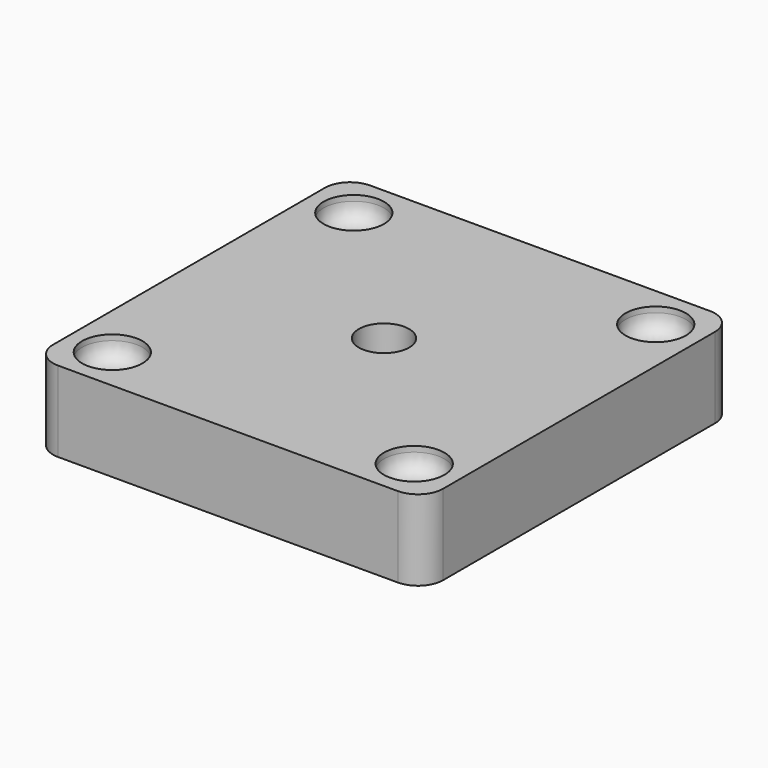
from build123d import *

# Parameters (mm, degrees)
F0_W         = 77.51
F0_H         = 77.519
F0_R         = 2.55
F0_R_2       = 5
F1_DEPTH     = 16
F2_DEPTH     = 7
F3_R         = 5
F4_R         = 6
F4_R_2       = 2.55
F5_DEPTH     = 4.6
F6_S5_R      = 2.55
F6_T6_DEPTH  = 10
F6_S11_R     = 2.55
F6_T12_DEPTH = 10
F6_S17_R     = 2.55
F6_T18_DEPTH = 10
F6_S23_R     = 2.55
F6_T24_DEPTH = 10


# Not quite as in the source:
# - a fillet or chamfer that OpenCascade refuses, or shapes differently, is made with other operations: its cross-section is extruded or revolved along the edge and cut away or added
# - a feature names something its author has since deleted; it is built from what else it names


with BuildPart() as f1:
    # F0 (on Top) → F1 (new body)
    with BuildSketch(Plane.XY):
        Rectangle(F0_W, F0_H)
        with Locations((-30, -29.9995)):
            Circle(F0_R, mode=Mode.SUBTRACT)
        with Locations((30, -29.9995)):
            Circle(F0_R, mode=Mode.SUBTRACT)
        with Locations((-30, 29.9995)):
            Circle(F0_R, mode=Mode.SUBTRACT)
        Polygon((7.25, -4.1857894516), (0, -8.3715789032), (-7.25, -4.1857894516), (-7.25, 4.1857894516), (0, 8.3715789032), (7.25, 4.1857894516), align=None, mode=Mode.SUBTRACT)
        with Locations((30, 29.9995)):
            Circle(F0_R, mode=Mode.SUBTRACT)
        Polygon((-7.25, -4.1857894516), (0, -8.3715789032), (7.25, -4.1857894516), (7.25, 4.1857894516), (0, 8.3715789032), (-7.25, 4.1857894516), align=None)
        Circle(F0_R_2, mode=Mode.SUBTRACT)
    extrude(amount=F1_DEPTH)

    # F0 (on Top) → F2 (cut)
    with BuildSketch(Plane.XY):
        Polygon((-7.25, -4.1857894516), (0, -8.3715789032), (7.25, -4.1857894516), (7.25, 4.1857894516), (0, 8.3715789032), (-7.25, 4.1857894516), align=None)
        Circle(F0_R_2, mode=Mode.SUBTRACT)
    extrude(amount=F2_DEPTH, mode=Mode.SUBTRACT)

    # F3
    f3_edges = [f1.edges().sort_by_distance(p)[0] for p in [
        (38.755, -38.7595, 8),
        (-38.755, -38.7595, 8),
        (38.755, 38.7595, 8),
        (-38.755, 38.7595, 8),
    ]]
    fillet(f3_edges, radius=F3_R)

    # F4 (on face) → F5 (cut)
    with BuildSketch(Plane.XY.offset(16)):
        with Locations((-30, 29.9995)):
            Circle(F4_R)
        with Locations((-30, 29.9995)):
            Circle(F4_R_2, mode=Mode.SUBTRACT)
        with Locations((30, 29.9995)):
            Circle(F4_R)
        with Locations((30, 29.9995)):
            Circle(F4_R_2, mode=Mode.SUBTRACT)
        with Locations((30, -29.9995)):
            Circle(F4_R)
        with Locations((30, -29.9995)):
            Circle(F4_R_2, mode=Mode.SUBTRACT)
        with Locations((-30, -29.9995)):
            Circle(F4_R)
        with Locations((-30, -29.9995)):
            Circle(F4_R_2, mode=Mode.SUBTRACT)
    extrude(amount=-F5_DEPTH, mode=Mode.SUBTRACT)

    # F6: fillet of radius 3.5 on 4 edges, made by hand


with BuildPart() as f6_tool2:
    # F6_s3 → F6_t4 (revolve)
    with BuildSketch(Plane.XZ.offset(29.9995)):
        with BuildLine():
            ThreePointArc((-24, 14.9), (-25.0251262658, 12.4251262658), (-27.5, 11.4))
            Line((-27.5, 11.4), (-24, 11.4))
            Line((-24, 11.4), (-24, 14.9))
        make_face()
    revolve(axis=Axis((-30, -29.9995, 11.4), (0, 0, 1)))

    # F6_s5 → F6_t6 (cut, symmetric)
    with BuildSketch(Plane.XY.offset(13.2)):
        with Locations((-30, -29.9995)):
            Circle(F6_S5_R)
    extrude(amount=F6_T6_DEPTH, both=True, mode=Mode.SUBTRACT)


with BuildPart() as f1_1:
    add(f1.part)

    # F6_t1: union F6_tool2
    add(f6_tool2.part)


with BuildPart() as f6_tool8:
    # F6_s9 → F6_t10 (revolve)
    with BuildSketch(Plane.XZ.offset(-29.9995)):
        with BuildLine():
            ThreePointArc((-24, 14.9), (-25.0251262658, 12.4251262658), (-27.5, 11.4))
            Line((-27.5, 11.4), (-24, 11.4))
            Line((-24, 11.4), (-24, 14.9))
        make_face()
    revolve(axis=Axis((-30, 29.9995, 11.4), (0, 0, 1)))

    # F6_s11 → F6_t12 (cut, symmetric)
    with BuildSketch(Plane.XY.offset(13.2)):
        with Locations((-30, 29.9995)):
            Circle(F6_S11_R)
    extrude(amount=F6_T12_DEPTH, both=True, mode=Mode.SUBTRACT)


with BuildPart() as f1_2:
    add(f1_1.part)

    # F6_t7: union F6_tool8
    add(f6_tool8.part)


with BuildPart() as f6_tool14:
    # F6_s15 → F6_t16 (revolve)
    with BuildSketch(Plane.XZ.offset(29.9995)):
        with BuildLine():
            ThreePointArc((36, 14.9), (34.9748737342, 12.4251262658), (32.5, 11.4))
            Line((32.5, 11.4), (36, 11.4))
            Line((36, 11.4), (36, 14.9))
        make_face()
    revolve(axis=Axis((30, -29.9995, 11.4), (0, 0, 1)))

    # F6_s17 → F6_t18 (cut, symmetric)
    with BuildSketch(Plane.XY.offset(13.2)):
        with Locations((30, -29.9995)):
            Circle(F6_S17_R)
    extrude(amount=F6_T18_DEPTH, both=True, mode=Mode.SUBTRACT)


with BuildPart() as f1_3:
    add(f1_2.part)

    # F6_t13: union F6_tool14
    add(f6_tool14.part)


with BuildPart() as f6_tool20:
    # F6_s21 → F6_t22 (revolve)
    with BuildSketch(Plane.XZ.offset(-29.9995)):
        with BuildLine():
            ThreePointArc((36, 14.9), (34.9748737342, 12.4251262658), (32.5, 11.4))
            Line((32.5, 11.4), (36, 11.4))
            Line((36, 11.4), (36, 14.9))
        make_face()
    revolve(axis=Axis((30, 29.9995, 11.4), (0, 0, 1)))

    # F6_s23 → F6_t24 (cut, symmetric)
    with BuildSketch(Plane.XY.offset(13.2)):
        with Locations((30, 29.9995)):
            Circle(F6_S23_R)
    extrude(amount=F6_T24_DEPTH, both=True, mode=Mode.SUBTRACT)


with BuildPart() as f1_4:
    add(f1_3.part)

    # F6_t19: union F6_tool20
    add(f6_tool20.part)


solid = f1_4.part
